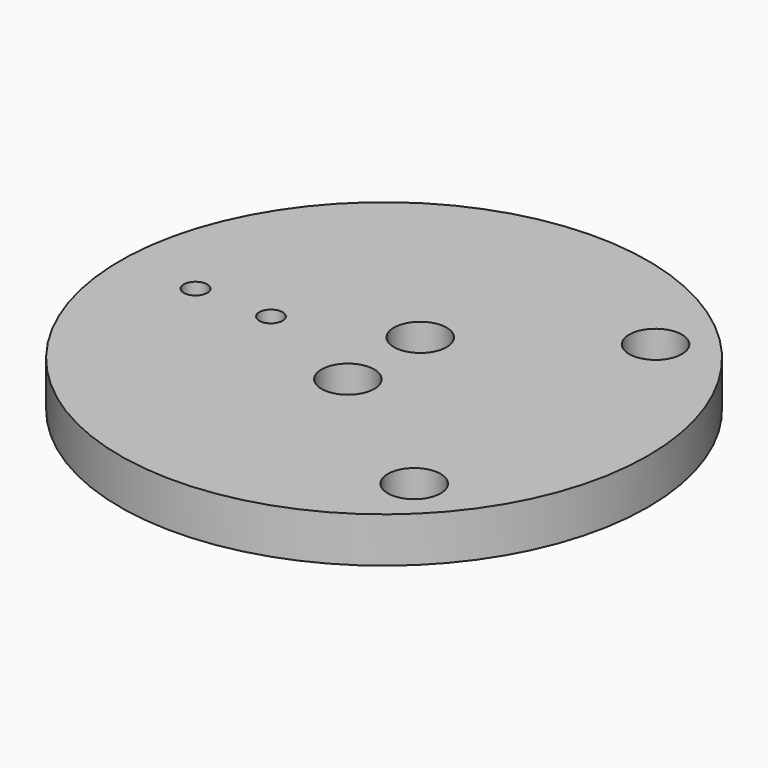
from build123d import *

# Parameters (mm, degrees)
F0_R     = 35
F1_DEPTH = 6
F2_R     = 1.55
F3_DEPTH = 6
F4_R     = 3.5
F4_R_2   = 1.55
F5_DEPTH = 4
F6_R     = 3.5
F7_DEPTH = 4


# Not quite as in the source:
# - a feature names something its author has since deleted; it is built from what else it names


with BuildPart() as f1:
    # F0 (on Top) → F1 (new body)
    with BuildSketch(Plane.XY):
        Circle(F0_R)
    extrude(amount=F1_DEPTH)

    # F2 (on face) → F3 (cut, through all)
    with BuildSketch(Plane.XY.offset(6)):
        with Locations((0, 6)):
            Circle(F2_R)
        with Locations((0, -6)):
            Circle(F2_R)
        with Locations((20, 20)):
            Circle(F2_R)
        with Locations((20, -20)):
            Circle(F2_R)
        with Locations((-15, 0)):
            Circle(F2_R)
        with Locations((-25, 0)):
            Circle(F2_R)
    extrude(amount=-F3_DEPTH, mode=Mode.SUBTRACT)

    # F4 (on face) → F5 (cut)
    with BuildSketch(Plane.XY.offset(6)):
        with Locations((0, -6)):
            Circle(F4_R)
        with Locations((0, 6)):
            Circle(F4_R)
        with Locations((20, -20)):
            Circle(F4_R)
        with Locations((20, 20)):
            Circle(F4_R)
        with Locations((20, 20)):
            Circle(F4_R_2)
        with Locations((20, -20)):
            Circle(F4_R_2)
    extrude(amount=-F5_DEPTH, mode=Mode.SUBTRACT)

    # F6 (on face) → F7 (cut)
    with BuildSketch(Plane(origin=(0, 0, 0), x_dir=(1, 0, 0), z_dir=(0, 0, -1))):
        with Locations((-25, 0)):
            Circle(F6_R)
        with Locations((-15, 0)):
            Circle(F6_R)
    extrude(amount=-F7_DEPTH, mode=Mode.SUBTRACT)


solid = f1.part
